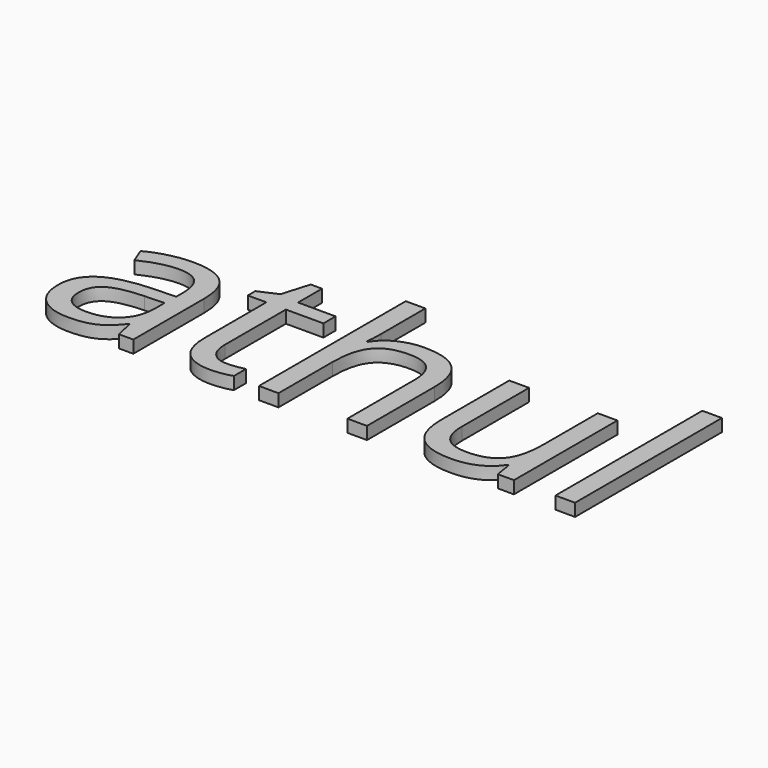
from build123d import *

# Parameters (mm, degrees)
F0_TEXT_SIZE = 490.2923686637
F1_DEPTH     = 25.4


# Not quite as in the source:
# - Text() gives the source's letters only with a copy of the font that has no kerning and outlines rounded to 1/6400 em; it was checked with that copy


with BuildPart() as f1:
    # F0 (on Top) → F1 (new body)
    with BuildSketch(Plane.XY):
        with Locations((-217.7140116692, -425.9826242924)):
            Text('athul', F0_TEXT_SIZE, font='Open Sans', text_align=(TextAlign.LEFT, TextAlign.BOTTOM))
    extrude(amount=F1_DEPTH)


solid = f1.part
